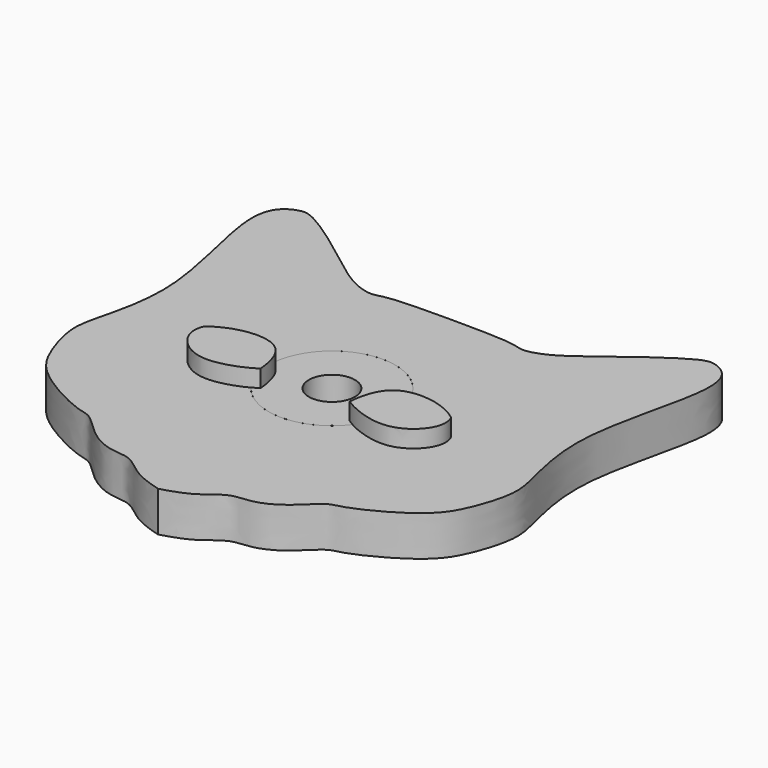
from build123d import *

# Parameters (mm, degrees)
F1_R     = 11
F1_R_2   = 4
F2_DEPTH = 7
F3_R     = 11
F4_DEPTH = 7
F6_DEPTH = 3


with BuildPart() as f2:
    # F1 (on Top) → F2 (new body)
    with BuildSketch(Plane.XY):
        Circle(F1_R)
        Circle(F1_R_2, mode=Mode.SUBTRACT)
    extrude(amount=F2_DEPTH)


with BuildPart() as f4:
    # F3 (on Top) → F4 (new body, through all)
    with BuildSketch(Plane.XY):
        with BuildLine():
            add(Edge.make_bspline(
                [(0, 25.8897617459), (4.3864055569, 25.8703153674), (10.8289101146, 25.8417536259), (13.2757002483, 24.6611704296), (17.8474108812, 26.2761901904), (23.594998976, 30.9202992901), (33.4937013261, 38.2138715063), (36.1675639167, 38.1806773323), (39.2855825143, 36.5848315949), (40.6715724711, 29.8977509674), (34.1473376422, 10.0883092219), (37.7336996012, -3.1394968098), (38.8698157184, -8.5086259705), (36.7537244866, -15.4845539707), (33.6701790157, -21.1369466388), (23.38847337, -26.5124231681), (20.5890565286, -26.5249775413), (17.1438835411, -30.5638448818), (12.6355944839, -33.0001390733), (8.5934381149, -32.6776161387), (5.0552641204, -36.2719007466), (1.7202712663, -37.2668030025), (0, -37.7799980342)],
                knots=[0, 0, 0, 0, 0.0656985275, 0.0964942838, 0.1366122657, 0.1933968461, 0.2619923062, 0.2926015893, 0.3258580246, 0.3741201394, 0.4650594165, 0.5378796558, 0.5831748819, 0.6344944194, 0.6862865162, 0.751805302, 0.784561497, 0.8284150022, 0.8732582997, 0.9115246968, 0.9543622644, 1, 1, 1, 1], degree=3))
            add(Edge.make_bspline(
                [(0, 25.8897617459), (-4.3864055569, 25.8703153674), (-10.8289101146, 25.8417536259), (-13.2757002483, 24.6611704296), (-17.8474108812, 26.2761901904), (-23.594998976, 30.9202992901), (-33.4937013261, 38.2138715063), (-36.1675639167, 38.1806773323), (-39.2855825143, 36.5848315949), (-40.6715724711, 29.8977509674), (-34.1473376422, 10.0883092219), (-37.7336996012, -3.1394968098), (-38.8698157184, -8.5086259705), (-36.7537244866, -15.4845539707), (-33.6701790157, -21.1369466388), (-23.38847337, -26.5124231681), (-20.5890565286, -26.5249775413), (-17.1438835411, -30.5638448818), (-12.6355944839, -33.0001390733), (-8.5934381149, -32.6776161387), (-5.0552641204, -36.2719007466), (-1.7202712663, -37.2668030025), (0, -37.7799980342)],
                knots=[0, 0, 0, 0, 0.0656985275, 0.0964942838, 0.1366122657, 0.1933968461, 0.2619923062, 0.2926015893, 0.3258580246, 0.3741201394, 0.4650594165, 0.5378796558, 0.5831748819, 0.6344944194, 0.6862865162, 0.751805302, 0.784561497, 0.8284150022, 0.8732582997, 0.9115246968, 0.9543622644, 1, 1, 1, 1], degree=3))
        make_face()
        Circle(F3_R, mode=Mode.SUBTRACT)
    extrude(amount=F4_DEPTH)

    # F5 (on face) → F6 (join)
    with BuildSketch(Plane.XY.offset(7)):
        with BuildLine():
            add(Edge.make_bspline(
                [(-21.2926585227, -1.0976089765), (-18.013806867, 1.4951896728), (-9.2317163321, 2.6104336842), (-7.8349251726, -3.4814778137), (-7.5953276828, -5.9909114283)],
                knots=[0, 0, 0, 0, 0.5514786848, 1, 1, 1, 1], degree=3))
            add(Edge.make_bspline(
                [(-21.2926585227, -1.0976089765), (-22.5738119334, -3.8589280234), (-18.404282887, -9.0247998666), (-12.0058316522, -8.2844709159), (-9.006950172, -6.913152259), (-7.5953276828, -5.9909114283)],
                knots=[0, 0, 0, 0, 0.3668386095, 0.6993561955, 1, 1, 1, 1], degree=3))
        make_face()
        with BuildLine():
            add(Edge.make_bspline(
                [(21.5854812413, -1.0976089765), (22.866634652, -3.8589280234), (18.6971056056, -9.0247998666), (12.2986543708, -8.2844709159), (9.2997728906, -6.913152259), (7.8881504014, -5.9909114283)],
                knots=[0, 0, 0, 0, 0.3668386095, 0.6993561955, 1, 1, 1, 1], degree=3))
            add(Edge.make_bspline(
                [(21.5854812413, -1.0976089765), (18.3066295856, 1.4951896728), (9.5245390508, 2.6104336842), (8.1277478912, -3.4814778137), (7.8881504014, -5.9909114283)],
                knots=[0, 0, 0, 0, 0.5514786848, 1, 1, 1, 1], degree=3))
        make_face()
    extrude(amount=F6_DEPTH)


solid = Compound([f2.part, f4.part])
